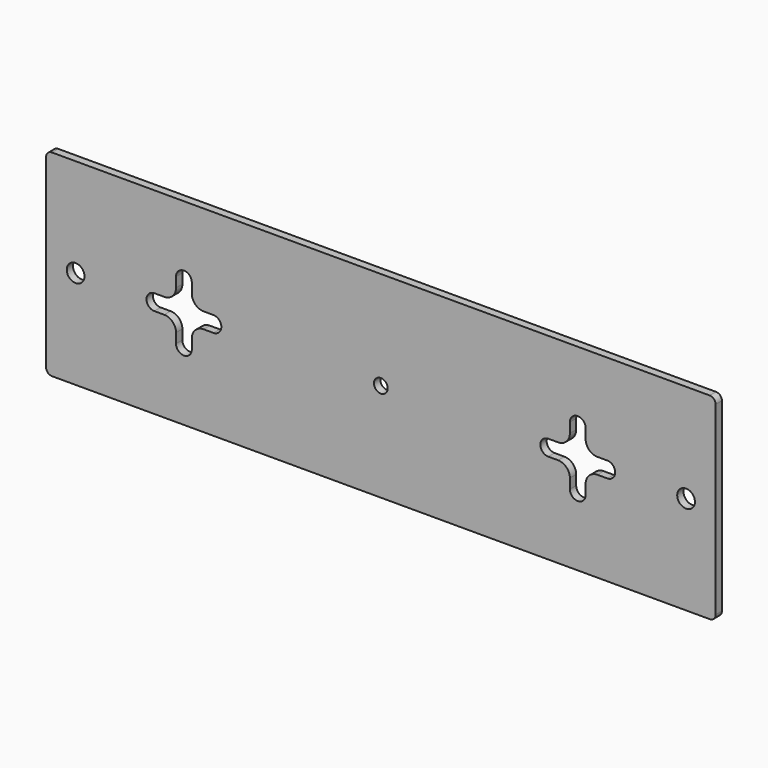
from build123d import *

# Parameters (mm, degrees)
F0_W     = 170
F0_H     = 50
F0_R     = 2.25
F0_R_2   = 1.75
F1_DEPTH = 2
F2_R     = 3
F3_R     = 1.5


# Not quite as in the source:
# - a feature names something its author has since deleted; it is built from what else it names


with BuildPart() as f1:
    # F0 (on Front) → F1 (new body)
    with BuildSketch(Plane.XZ):
        with Locations((85, 25)):
            Rectangle(F0_W, F0_H)
        with Locations((7.5, 25)):
            Circle(F0_R, mode=Mode.SUBTRACT)
        with BuildLine():
            Line((27.5, 27), (33, 27))
            Line((33, 27), (33, 32.5))
            ThreePointArc((33, 32.5), (35, 34.5), (37, 32.5))
            Line((37, 32.5), (37, 27))
            Line((37, 27), (42.5, 27))
            ThreePointArc((42.5, 27), (44.5, 25), (42.5, 23))
            Line((42.5, 23), (37, 23))
            Line((37, 23), (37, 17.5))
            ThreePointArc((37, 17.5), (35, 15.5), (33, 17.5))
            Line((33, 17.5), (33, 23))
            Line((33, 23), (27.5, 23))
            ThreePointArc((27.5, 23), (25.5, 25), (27.5, 27))
        make_face(mode=Mode.SUBTRACT)
        with Locations((85, 25)):
            Circle(F0_R_2, mode=Mode.SUBTRACT)
        with BuildLine():
            ThreePointArc((127.5, 23), (125.5, 25), (127.5, 27))
            Line((127.5, 27), (133, 27))
            Line((133, 27), (133, 32.5))
            ThreePointArc((133, 32.5), (135, 34.5), (137, 32.5))
            Line((137, 32.5), (137, 27))
            Line((137, 27), (142.5, 27))
            ThreePointArc((142.5, 27), (144.5, 25), (142.5, 23))
            Line((142.5, 23), (137, 23))
            Line((137, 23), (137, 17.5))
            ThreePointArc((137, 17.5), (135, 15.5), (133, 17.5))
            Line((133, 17.5), (133, 23))
            Line((133, 23), (127.5, 23))
        make_face(mode=Mode.SUBTRACT)
        with Locations((162.5, 25)):
            Circle(F0_R, mode=Mode.SUBTRACT)
    extrude(amount=F1_DEPTH)

    # F2
    f2_edges = [f1.edges().sort_by_distance(p)[0] for p in [
        (33, -1, 27),
        (37, -1, 27),
        (37, -1, 23),
        (33, -1, 23),
        (133, -1, 27),
        (133, -1, 23),
        (137, -1, 27),
        (137, -1, 23),
    ]]
    fillet(f2_edges, radius=F2_R)

    # F3
    f3_edges = [f1.edges().sort_by_distance(p)[0] for p in [
        (0, -1, 50),
        (0, -1, 0),
        (170, -1, 50),
        (170, -1, 0),
    ]]
    fillet(f3_edges, radius=F3_R)


solid = f1.part
